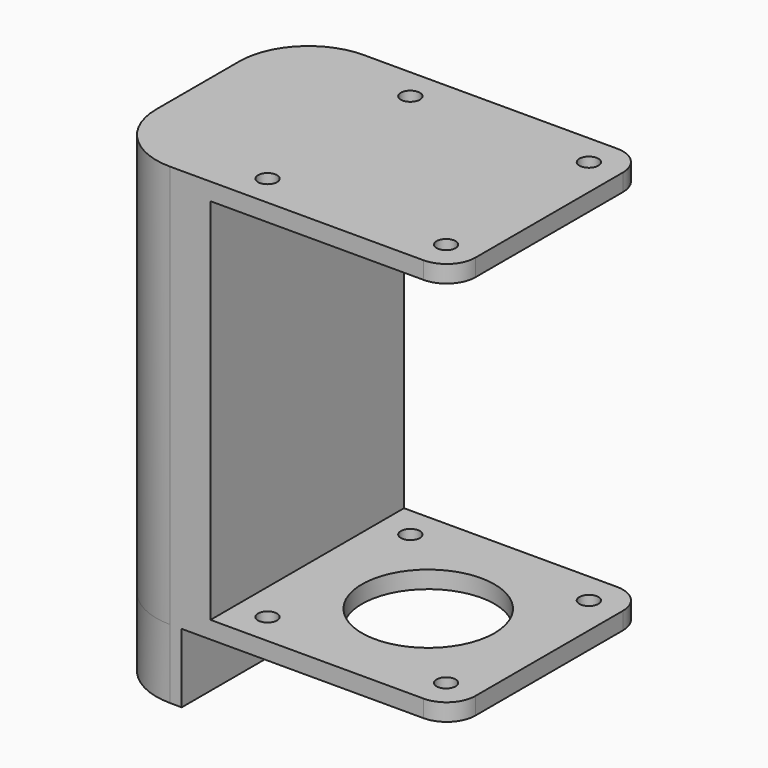
from build123d import *

# Parameters (mm, degrees)
F0_W      = 42
F0_H      = 42
F1_DEPTH  = 3
F2_R      = 11.5
F3_DEPTH  = 25
F4_W      = 42
F4_H      = 3
F4_H_2    = 67
F5_DEPTH  = 19
F6_W      = 42
F6_H      = 3
F7_DEPTH  = 42
F8_R      = 5
F9_D      = 3.3
F10_R     = 12
F12_DEPTH = 12
F14_DEPTH = 1


# Not quite as in the source:
# - a feature names something its author has since deleted; it is built from what else it names


with BuildPart() as f1:
    # F0 (on Top) → F1 (new body)
    with BuildSketch(Plane.XY):
        Rectangle(F0_W, F0_H)
    extrude(amount=F1_DEPTH)

    # F2 (on face) → F3 (cut)
    with BuildSketch(Plane(origin=(0, 0, 0), x_dir=(1, 0, 0), z_dir=(0, 0, -1))):
        Circle(F2_R)
    extrude(amount=-F3_DEPTH, mode=Mode.SUBTRACT)

    # F4 (on face) → F5 (join)
    with BuildSketch(Plane(origin=(-21, 0, 0), x_dir=(0, -1, 0), z_dir=(-1, 0, 0))):
        with Locations((0, 1.5)):
            Rectangle(F4_W, F4_H)
        with Locations((0, 36.5)):
            Rectangle(F4_W, F4_H_2)
    extrude(amount=F5_DEPTH)

    # F6 (on face) → F7 (join)
    with BuildSketch(Plane.YZ.offset(-21)):
        with Locations((0, 68.5)):
            Rectangle(F6_W, F6_H)
    extrude(amount=F7_DEPTH)

    # F8
    f8_edges = [f1.edges().sort_by_distance(p)[0] for p in [
        (21, 21, 1.5),
        (21, -21, 1.5),
        (21, -21, 68.5),
        (21, 21, 68.5),
    ]]
    fillet(f8_edges, radius=F8_R)

    # F9 (through all)
    with Locations(Plane(origin=(0, 0, 0), x_dir=(1, 0, 0), z_dir=(0, 0, -1))):
        with Locations((-15.5, -15.5), (15.5, -15.5), (15.5, 15.5), (-15.5, 15.5)):
            Hole(F9_D / 2)

    # F10
    f10_edges = [f1.edges().sort_by_distance(p)[0] for p in [
        (-40, -21, 35),
        (-40, 21, 35),
    ]]
    fillet(f10_edges, radius=F10_R)

    # F11 (on face) → F12 (join)
    with BuildSketch(Plane(origin=(0, 0, 0), x_dir=(1, 0, 0), z_dir=(0, 0, -1))):
        with BuildLine():
            Line((-26, -21), (-26, 21))
            Line((-26, 21), (-28, 21))
            ThreePointArc((-28, 21), (-36.4852813742, 17.4852813742), (-40, 9))
            Line((-40, 9), (-40, -9))
            ThreePointArc((-40, -9), (-36.4852813742, -17.4852813742), (-28, -21))
            Line((-28, -21), (-26, -21))
        make_face()
    extrude(amount=F12_DEPTH)

    # F13 (on face) → F14 (cut)
    with BuildSketch(Plane(origin=(0, 0, -12), x_dir=(1, 0, 0), z_dir=(0, 0, -1))):
        Polygon((-34.3291561734, 13.8271097128), (-34.3291561734, 13.8010392968), (-34.3163219754, 13.7125962563), (-34.2802923934, 13.6341532066), (-34.2247797128, 13.5694196654), (-34.1534948353, 13.5221079183), (-34.0701486625, 13.4959288669), (-33.9744900184, 13.4918830639), (-33.6002328215, 13.4918830639), (-32.9923355135, 13.4918830639), (-32.3260283508, 13.4918830639), (-31.7765408976, 13.4918830639), (-31.5191041022, 13.4918830639), (-31.7002456455, 13.3605228197), (-32.2358187745, 12.9783905954), (-32.9383236619, 12.477151783), (-33.6199622525, 11.9908008617), (-34.092935799, 11.6533336945), (-34.2138622028, 11.5664143172), (-34.2522084171, 11.5296983256), (-34.2834206772, 11.4874177114), (-34.3069654936, 11.4406069325), (-34.3223107603, 11.3902976792), (-34.3289257556, 11.3375257932), (-34.3291561734, 11.3008194889), (-34.3291561734, 11.2133846124), (-34.3291561734, 11.093462221), (-34.3291561734, 10.9735405215), (-34.3291561734, 10.8861056451), (-34.3284988255, 10.8410323404), (-34.3101892659, 10.7545011443), (-34.2695091207, 10.678789202), (-34.2101706756, 10.6176101828), (-34.1358848322, 10.5746756805), (-34.050363184, 10.5536972886), (-33.8706491234, 10.5522255213), (-33.2083116497, 10.5522255213), (-32.2537657549, 10.5522255213), (-31.2699997098, 10.5522255213), (-30.5199997098, 10.5522255213), (-30.2519789219, 10.5523908962), (-30.1644693154, 10.5679852632), (-30.0873617198, 10.6063619231), (-30.0243718803, 10.6638078983), (-29.9792148503, 10.7366102114), (-29.955606375, 10.8210579608), (-29.9530025855, 10.8704510788), (-29.9530025855, 10.9234865959), (-29.9530025855, 11.0043016334), (-29.9530025855, 11.0901678703), (-29.9530025855, 11.1583556015), (-29.9530025855, 11.1861365058), (-29.9658409352, 11.274569859), (-30.0018795125, 11.3530115248), (-30.0574025722, 11.4177478338), (-30.1286943692, 11.4650637326), (-30.21203985, 11.4912455518), (-30.3080562297, 11.4952927387), (-30.6852977859, 11.4952927387), (-31.2980428613, 11.4952927387), (-31.9696641626, 11.4952927387), (-32.5235330122, 11.4952927387), (-32.7830228088, 11.4952927387), (-32.6006191575, 11.6262302044), (-32.0613046814, 12.007134918), (-31.3538918273, 12.5067635742), (-30.6674912704, 12.9915513915), (-30.191212994, 13.3279349727), (-30.0694161233, 13.4145976383), (-30.0307197848, 13.4513419997), (-29.9992086043, 13.4937326331), (-29.9754278347, 13.5407212419), (-29.9599220367, 13.5912574532), (-29.953235771, 13.6442915864), (-29.9530025855, 13.6802755001), (-29.9530025855, 13.764942596), (-29.9530025855, 13.8810682846), (-29.9530025855, 13.9971946652), (-29.9530025855, 14.0818617612), (-29.9536599334, 14.1261538598), (-29.9719757205, 14.2126954351), (-30.012664861, 14.288412913), (-30.0720136852, 14.3495953918), (-30.1463050643, 14.39253197), (-30.2318239447, 14.4135103619), (-30.4115338536, 14.4149821292), (-31.0738713272, 14.4149821292), (-32.0284172221, 14.4149821292), (-33.0121839591, 14.4149821292), (-33.7621839591, 14.4149821292), (-34.0302054389, 14.4148167543), (-34.117720581, 14.3992216953), (-34.1948240249, 14.3608443435), (-34.2578048691, 14.3033956005), (-34.30295152, 14.2305877518), (-34.3265530758, 14.1461310072), (-34.3291561734, 14.0972921372), (-34.3291561734, 14.0475212172), (-34.3291561734, 13.971680573), (-34.3291561734, 13.8911001049), align=None)
        Polygon((-32.3764234053, 5.4123437425), (-32.1428005929, 5.4026316009), (-31.9076015295, 5.4119943102), (-31.6828113965, 5.440083822), (-31.4684281179, 5.4869022123), (-31.2644482342, 5.5524515567), (-31.0708689774, 5.6367332393), (-30.8876882718, 5.7397486438), (-30.7149026576, 5.8615012301), (-30.5525107509, 6.001992382), (-30.4038726373, 6.1579222132), (-30.2743619624, 6.3241717138), (-30.164045845, 6.5006813766), (-30.0729222092, 6.6874491257), (-30.0009869033, 6.8844721933), (-29.9482385434, 7.0917491955), (-29.9146736699, 7.3092780566), (-29.9002895149, 7.5370567006), (-29.9051123723, 7.7694139454), (-29.9292121286, 7.9925081209), (-29.9725950114, 8.2057102492), (-30.0352651722, 8.4090182542), (-30.1172260709, 8.6024293684), (-30.2184811671, 8.7859422076), (-30.3390339205, 8.9595546962), (-30.4788884829, 9.1232633744), (-30.6361772943, 9.2753113936), (-30.8040092734, 9.4089329143), (-30.9817422951, 9.5234602097), (-31.1693749756, 9.6188946636), (-31.3669059309, 9.6952383518), (-31.5743330853, 9.7524933502), (-31.7916543628, 9.7906617346), (-32.0188683795, 9.8097448889), (-32.254293709, 9.809718595), (-32.4828992274, 9.7904271652), (-32.701353911, 9.7518456896), (-32.9096591436, 9.693976244), (-33.1078135415, 9.6168202122), (-33.2958184885, 9.5203796701), (-33.4736732925, 9.4046566935), (-33.6413779538, 9.2696533584), (-33.7982751243, 9.1160110977), (-33.9376944531, 8.9503912671), (-34.0578950065, 8.7745610944), (-34.1588733246, 8.5885247313), (-34.2406259478, 8.3922884053), (-34.3031487243, 8.1858548842), (-34.3464381945, 7.9692303954), (-34.3704902066, 7.7424183987), (-34.3753040688, 7.5117128269), (-34.360955203, 7.3005567804), (-34.3274733628, 7.0966059583), (-34.2748557806, 6.8998672801), (-34.2031017643, 6.7103469734), (-34.1122078543, 6.5280519575), (-34.0021733585, 6.35298846), (-33.8729962012, 6.1851634003), (-33.7247441929, 6.0246605039), (-33.5628484109, 5.8788213082), (-33.3907208365, 5.7524472205), (-33.2083545503, 5.6455327053), (-33.0157467845, 5.5580715349), (-32.8128920035, 5.490057482), (-32.5997860556, 5.4414829351), align=None)
        Polygon((-33.4991237257, 7.4768816938), (-33.5027460584, 7.6090044615), (-33.4947935332, 7.7410372763), (-33.4759456403, 7.8664730864), (-33.4461996118, 7.9853056643), (-33.4055540639, 8.0975322421), (-33.3540062288, 8.2031472845), (-33.2915547227, 8.3021466396), (-33.2181967776, 8.3945254639), (-33.1339296259, 8.4802796056), (-33.0401980489, 8.5581379617), (-32.939166451, 8.6259651894), (-32.8308555906, 8.6837329191), (-32.7152661594, 8.7314439186), (-32.5923967737, 8.7691030314), (-32.4622488174, 8.7967137172), (-32.3248209066, 8.8142815117), (-32.1801144251, 8.8218084906), (-32.0304051804, 8.8192406823), (-31.8869573471, 8.8064334702), (-31.7508358286, 8.7833813188), (-31.6220371653, 8.750083536), (-31.5005599731, 8.706540814), (-31.3864007926, 8.6527517687), (-31.2795582396, 8.588717784), (-31.1800288545, 8.5144381681), (-31.0886222131, 8.4306173209), (-31.0083870256, 8.3401046727), (-30.9396146008, 8.2431963757), (-30.8823049388, 8.1398868945), (-30.8364573475, 8.0301686176), (-30.802072519, 7.9140367015), (-30.7791497613, 7.7914835347), (-30.7676883825, 7.6625042737), (-30.767706373, 7.5319017095), (-30.7793151362, 7.4085728722), (-30.8025354303, 7.2906799558), (-30.8373679473, 7.1782278038), (-30.8838161469, 7.0712205679), (-30.941882105, 6.9696630917), (-31.0115672054, 6.8735602189), (-31.0928749078, 6.782916101), (-31.1853893533, 6.6980829382), (-31.2850190704, 6.6226913665), (-31.3907226817, 6.5577052653), (-31.5024974195, 6.5031211751), (-31.6203391319, 6.4589384038), (-31.7442436675, 6.4251548756), (-31.8742082584, 6.4017678227), (-32.0102294448, 6.3887765532), (-32.1539388334, 6.3861720718), (-32.3005384767, 6.3938201411), (-32.4402781762, 6.4116647137), (-32.5731572399, 6.4397057894), (-32.699172208, 6.4779433683), (-32.8183230807, 6.5263774503), (-32.9306077819, 6.5850080356), (-33.036024928, 6.6538351241), (-33.1345364618, 6.7328310379), (-33.2229760425, 6.8197386521), (-33.2992948207, 6.9131111096), (-33.3634941802, 7.0129463344), (-33.415575505, 7.1192436346), (-33.455539487, 7.2319995505), (-33.4833888939, 7.3512126982), align=None, mode=Mode.SUBTRACT)
        Polygon((-34.1037571286, 1.8411790328), (-34.0199999404, 1.8296982794), (-33.731121851, 1.8296982794), (-33.0121839591, 1.8296982794), (-32.0847318671, 1.8296982794), (-31.1703118693, 1.8296982794), (-30.4904702602, 1.8296982794), (-30.2519789219, 1.8298636543), (-30.1690928927, 1.843962728), (-30.0953004061, 1.8785696708), (-30.0337325138, 1.9305561991), (-29.9875181917, 1.9967954129), (-29.9597884912, 2.0741583362), (-29.9530025855, 2.140396858), (-29.9530025855, 2.1758507417), (-29.9530025855, 2.2439858851), (-29.9530025855, 2.3256437117), (-29.9530025855, 2.4016670294), (-29.9530025855, 2.4528979536), (-29.9544750447, 2.4941870104), (-29.9736834411, 2.5752096315), (-30.012664861, 2.6463962528), (-30.0682896366, 2.7046213582), (-30.1374281004, 2.746755972), (-30.2169485086, 2.769674578), (-30.2873387011, 2.7729606254), (-30.4784317991, 2.7729606254), (-30.789516483, 2.7729606254), (-31.1389985852, 2.7729606254), (-31.4452839378, 2.7729606254), (-31.6267776812, 2.7729606254), (-31.6461729027, 2.7920949836), (-31.6461729027, 2.8167524477), (-31.6461729027, 2.8436303637), (-31.6461729027, 2.8788842752), (-31.5843365358, 2.921018889), (-31.3295208284, 3.0914601931), (-30.9613942652, 3.3376916294), (-30.57168455, 3.5983605004), (-30.2521200787, 3.8121106492), (-30.0944271713, 3.9175879945), (-30.0563369768, 3.9466496892), (-30.0209149225, 3.9839988106), (-29.9923638833, 4.0263797568), (-29.9711931306, 4.0728424873), (-29.9579084764, 4.1224376532), (-29.9530178083, 4.1742152141), (-29.9530025855, 4.2005554887), (-29.9530025855, 4.2636539636), (-29.9530025855, 4.3467282019), (-29.9530025855, 4.4298024403), (-29.9530025855, 4.4929009151), (-29.953084927, 4.5235388608), (-29.9778150453, 4.6389117131), (-30.0395939809, 4.7311417692), (-30.1281996284, 4.7947792693), (-30.2334098829, 4.8243779135), (-30.345002639, 4.8144893259), (-30.4380242803, 4.7704608583), (-30.574143723, 4.6790985014), (-30.8499883342, 4.4939512878), (-31.1863816026, 4.2681647538), (-31.5041449408, 4.0548830519), (-31.7240997614, 3.9072496425), (-31.7985212261, 3.9177519855), (-31.8759228984, 4.0642374578), (-31.9623641416, 4.1936664832), (-32.0578511833, 4.3060259145), (-32.162390251, 4.4013039888), (-32.2759868802, 4.479488943), (-32.3977415423, 4.5411689304), (-32.5197812858, 4.5915155487), (-32.6402828353, 4.6317230954), (-32.7592489586, 4.6617964139), (-32.8766858832, 4.6817417318), (-32.9925963768, 4.6915625087), (-33.1507944042, 4.6895876974), (-33.3368169283, 4.6668524568), (-33.5087735923, 4.622033096), (-33.6666685476, 4.5551309989), (-33.8105080219, 4.4661468573), (-33.9402961668, 4.3550834392), (-34.0547826374, 4.2232125395), (-34.1496040279, 4.0750491002), (-34.2243915316, 3.9109868381), (-34.2791506839, 3.7310195256), (-34.3138856367, 3.5351409352), (-34.3286026173, 3.3233469153), (-34.3291561734, 3.2187656389), (-34.3291561734, 3.0266180166), (-34.3291561734, 2.7559318561), (-34.3291561734, 2.4734660221), (-34.3291561734, 2.2459759192), (-34.3291561734, 2.1402197201), (-34.320171958, 2.0645811239), (-34.2901131703, 1.9883647536), (-34.2419406435, 1.9236402077), (-34.1787798936, 1.8735357701), align=None)
        Polygon((-33.5022104929, 2.7795756206), (-33.5492966659, 2.7795756206), (-33.5492966659, 2.8123122359), (-33.5492966659, 2.846046636), (-33.5492966659, 2.8849713164), (-33.5492966659, 2.9242952491), (-33.5492966659, 2.9592274062), (-33.5492966659, 2.9967543574), (-33.5477868417, 3.0650894729), (-33.5419890335, 3.1426841979), (-33.5318430424, 3.2158207205), (-33.5173474842, 3.2844976569), (-33.498503051, 3.348714315), (-33.4753097427, 3.4084679272), (-33.4477661756, 3.4637584934), (-33.4158730414, 3.5145839378), (-33.3799223411, 3.5606647146), (-33.3408648073, 3.6010466314), (-33.2987696344, 3.6356549581), (-33.2536312869, 3.6644903868), (-33.205446305, 3.6875543014), (-33.1542091533, 3.7048501614), (-33.099914988, 3.7163786589), (-33.0425603496, 3.7221418698), (-32.9411170443, 3.7200916364), (-32.8114569093, 3.6979265586), (-32.6998932148, 3.653595711), (-32.6064259609, 3.5870984018), (-32.5310516878, 3.4984318631), (-32.4737703955, 3.3875967868), (-32.4345793162, 3.2545917891), (-32.4134777581, 3.0994147941), (-32.4094582489, 2.9691028468), (-32.4094582489, 2.9431888104), (-32.4094582489, 2.9094059742), (-32.4094582489, 2.8722519813), (-32.4094582489, 2.8362217073), (-32.4094582489, 2.8058107196), (-32.4108628975, 2.7795756206), (-32.4725982405, 2.7795756206), (-32.6075780495, 2.7795756206), (-32.7906895606, 2.7795756206), (-32.9968213937, 2.7795756206), (-33.2008607848, 2.7795756206), (-33.3776942778, 2.7795756206), align=None, mode=Mode.SUBTRACT)
        Polygon((-34.3291561734, -1.2968889273), (-34.3291561734, -1.4208239085), (-34.3213088238, -1.4903464018), (-34.2989313189, -1.5543188033), (-34.263769436, -1.6109946436), (-34.2175703366, -1.6586288371), (-34.1620784144, -1.6954742225), (-34.0990415227, -1.7197850221), (-34.0302054389, -1.7298154584), (-34.0076168907, -1.7299801414), (-33.9677656958, -1.7299801414), (-33.91032664, -1.7299801414), (-33.8455591936, -1.7299801414), (-33.7837235185, -1.7299801414), (-33.7350777012, -1.7299801414), (-33.7098825958, -1.7299801414), (-33.6582849406, -1.7259343383), (-33.5925563824, -1.7075299822), (-33.5336220332, -1.6758423557), (-33.4832297465, -1.6326186203), (-33.4431252997, -1.5796038616), (-33.4150551623, -1.518544549), (-33.4007671876, -1.451187152), (-33.3992954204, -1.4083294556), (-33.3992954204, -1.3356503087), (-33.3992954204, -1.2177006527), (-33.3992954204, -1.0771153963), (-33.3992954204, -0.9365301399), (-33.3992954204, -0.8185797921), (-33.3992954204, -0.7459006452), (-33.3667698484, -0.7334061923), (-33.0730356882, -0.7334061923), (-32.5579469024, -0.7334061923), (-31.9248025931, -0.7334061923), (-31.2769011704, -0.7334061923), (-30.7175410443, -0.7334061923), (-30.3500220089, -0.7334061923), (-30.2418578408, -0.7327488444), (-30.1737469155, -0.7205713024), (-30.1116794389, -0.6943624973), (-30.0574025722, -0.6558668229), (-30.012664861, -0.6068307486), (-29.9792148503, -0.5490000519), (-29.9588003936, -0.4841205103), (-29.9530025855, -0.4238375601), (-29.9530025855, -0.4019298859), (-29.9530025855, -0.3540389807), (-29.9530025855, -0.2908636999), (-29.9530025855, -0.2231028989), (-29.9530025855, -0.1614561249), (-29.9530025855, -0.0993000793), (-29.9608520109, -0.029776894), (-29.9832357434, 0.0341989672), (-30.0184059296, 0.0908796512), (-30.0646133323, 0.1385186883), (-30.1201100981, 0.1753689173), (-30.1831483737, 0.1996838685), (-30.2519789219, 0.2097149968), (-30.3868646264, 0.2098803717), (-30.7881139103, 0.2098803717), (-31.3664464794, 0.2098803717), (-32.0185646156, 0.2098803717), (-32.641168525, 0.2098803717), (-33.1309591055, 0.2098803717), (-33.384638639, 0.2098803717), (-33.3992954204, 0.2293129583), (-33.3992954204, 0.310617201), (-33.3992954204, 0.4343618973), (-33.3992954204, 0.5776941758), (-33.3992954204, 0.7177618572), (-33.3992954204, 0.8317127623), (-33.3992954204, 0.8966940198), (-33.4018985179, 0.944194668), (-33.4182623279, 1.0107618637), (-33.4481578165, 1.0707825667), (-33.4898392062, 1.1225109994), (-33.5415586437, 1.1641986167), (-33.6015710433, 1.1940996408), (-33.6681278599, 1.2104662186), (-33.711657435, 1.213070008), (-33.7408305329, 1.213070008), (-33.7919888029, 1.213070008), (-33.8548713909, 1.213070008), (-33.9192202106, 1.213070008), (-33.9747744079, 1.213070008), (-34.0112758965, 1.213070008), (-34.040327904, 1.2124126602), (-34.1084429809, 1.2002337343), (-34.1705083817, 1.1740214695), (-34.2247797128, 1.1355230273), (-34.2695091207, 1.0864848771), (-34.30295152, 1.0286548723), (-34.3233604411, 0.9637794824), (-34.3291561734, 0.9011369994), (-34.3291561734, 0.7443955166), (-34.3291561734, 0.401751216), (-34.3291561734, -0.0502473982), (-34.3291561734, -0.5350525142), (-34.3291561734, -0.9761156279), align=None)
        Polygon((-34.3291561734, -5.4243000101), (-34.3291561734, -5.4537692605), (-34.3148944926, -5.5468573285), (-34.2750183877, -5.6285822738), (-34.2138940323, -5.694576539), (-34.1358848322, -5.7404718745), (-34.0453569611, -5.7619007227), (-33.8829678222, -5.7629254934), (-33.3650005447, -5.7629254934), (-32.6577406105, -5.7629254934), (-31.9727502378, -5.7629254934), (-31.5215923368, -5.7629254934), (-31.3504376373, -5.7595529529), (-31.1437889212, -5.7302781391), (-30.9408718651, -5.6709230873), (-30.7417037676, -5.5814725747), (-30.5463005435, -5.4619113786), (-30.3553707446, -5.3121426267), (-30.1904656933, -5.1290497981), (-30.0618019593, -4.9110642533), (-29.9693691633, -4.6581873762), (-29.9131555423, -4.3704219345), (-29.8931493332, -4.0477679283), (-29.8999995899, -3.8541097897), (-29.9222656917, -3.6753063289), (-29.9599365675, -3.5033579683), (-30.0130308999, -3.3382723193), (-30.0815673714, -3.1800563015), (-30.1650560849, -3.0306155315), (-30.2621982593, -2.8957997134), (-30.3729364632, -2.776028166), (-30.4972727726, -2.6713071168), (-30.6352127228, -2.5816434852), (-30.7853717318, -2.5069424746), (-30.9361036713, -2.4463516089), (-31.0847853775, -2.399692366), (-31.2314189261, -2.3669772011), (-31.3760036253, -2.3482213368), (-31.5028496195, -2.343264242), (-31.808884488, -2.343264242), (-32.4210490215, -2.343264242), (-33.1316123017, -2.343264242), (-33.7328441024, -2.343264242), (-34.0170121215, -2.343264242), (-34.1037571286, -2.3547429195), (-34.1868867225, -2.392128022), (-34.2547395523, -2.4512222105), (-34.30295152, -2.5276593113), (-34.3271585278, -2.6170752266), (-34.3291561734, -2.6646755148), (-34.3291561734, -2.7229462886), (-34.3291561734, -2.8065962253), (-34.3291561734, -2.890246162), (-34.3291561734, -2.9485162438), (-34.3271585278, -2.996117224), (-34.30295152, -3.0855331393), (-34.2547395523, -3.1619702401), (-34.1868867225, -3.2210637366), (-34.1037571286, -3.2584488392), (-34.0172529184, -3.2699275166), (-33.7559792873, -3.2699275166), (-33.2031871042, -3.2699275166), (-32.5498719029, -3.2699275166), (-31.9870278332, -3.2699275166), (-31.7056497369, -3.2699275166), (-31.5710062132, -3.2753800441), (-31.4309150056, -3.2960242266), (-31.3044149839, -3.3320600361), (-31.1915192951, -3.38349716), (-31.0922410861, -3.4503439015), (-31.007058491, -3.5321657192), (-30.938087478, -3.6267705309), (-30.8855909861, -3.7338670277), (-30.849574551, -3.8534628211), (-30.8300437083, -3.9855634465), (-30.8269991498, -4.1230806183), (-30.840359918, -4.2433302997), (-30.8700921075, -4.354190286), (-30.9161901829, -4.4556591932), (-30.9786486085, -4.5477384053), (-31.0574521616, -4.6304258463), (-31.1494178947, -4.7007606831), (-31.2519724638, -4.7561474297), (-31.365115177, -4.7965957732), (-31.4888453424, -4.8221133251), (-31.623162268, -4.8327097726), (-31.7965962348, -4.8330405223), (-32.2876558426, -4.8330405223), (-32.9427908595, -4.8330405223), (-33.5671619968, -4.8330405223), (-33.9659285815, -4.8330405223), (-34.0701486625, -4.8370863254), (-34.1578056533, -4.8653737336), (-34.2317946523, -4.9169769243), (-34.2877508697, -4.9875324916), (-34.3213088238, -5.072674262), (-34.3291561734, -5.1444552641), (-34.3291561734, -5.1874222878), (-34.3291561734, -5.265481308), (-34.3291561734, -5.3529895306), align=None)
        Polygon((-34.3291561734, -8.5249925549), (-34.3291561734, -8.7168633992), (-34.3133964315, -8.8145736605), (-34.2695091207, -8.8994393447), (-34.2025869572, -8.96636566), (-34.117720581, -9.0102571224), (-34.0199999404, -9.0260196321), (-33.6291872648, -9.0260196321), (-32.6972486006, -9.0260196321), (-31.5849343763, -9.0260196321), (-30.6529957122, -9.0260196321), (-30.2621830365, -9.0260196321), (-30.1644693154, -9.0102571224), (-30.0795980956, -8.96636566), (-30.012664861, -8.8994393447), (-29.968767171, -8.8145736605), (-29.9530025855, -8.7168633992), (-29.9530025855, -8.5249925549), (-29.9530025855, -8.0674556119), (-29.9530025855, -7.5213628414), (-29.9530025855, -7.0638252066), (-29.9530025855, -6.8719550542), (-29.968767171, -6.7742337217), (-30.012664861, -6.68936181), (-30.0795980956, -6.622432727), (-30.1644693154, -6.5785405726), (-30.2621830365, -6.562777371), (-30.2880015845, -6.562777371), (-30.3495680929, -6.562777371), (-30.4230505881, -6.562777371), (-30.4846170964, -6.562777371), (-30.5104356444, -6.562777371), (-30.60814383, -6.5785405726), (-30.6930032867, -6.622432727), (-30.7599219905, -6.68936181), (-30.8038072254, -6.7742337217), (-30.8195676593, -6.8719550542), (-30.8195676593, -6.9978759178), (-30.8195676593, -7.2981489594), (-30.8195676593, -7.6565391629), (-30.8195676593, -7.9568122044), (-30.8195676593, -8.0827330681), (-30.9138458729, -8.0827330681), (-31.1386643757, -8.0827330681), (-31.4069958469, -8.0827330681), (-31.6318136578, -8.0827330681), (-31.7260925633, -8.0827330681), (-31.7260925633, -7.9568122044), (-31.7260925633, -7.6565391629), (-31.7260925633, -7.2981489594), (-31.7260925633, -6.9978759178), (-31.7260925633, -6.8719550542), (-31.741855073, -6.7742337217), (-31.7857465354, -6.68936181), (-31.8526721587, -6.622432727), (-31.9375378429, -6.5785405726), (-32.0352487962, -6.562777371), (-32.0596931412, -6.562777371), (-32.1179846734, -6.562777371), (-32.1875590625, -6.562777371), (-32.2458505947, -6.562777371), (-32.2702949397, -6.562777371), (-32.3680176561, -6.5785405726), (-32.4528909517, -6.622432727), (-32.5198200347, -6.68936181), (-32.563712881, -6.7742337217), (-32.5794760826, -6.8719550542), (-32.5794760826, -6.9978759178), (-32.5794760826, -7.2981489594), (-32.5794760826, -7.6565391629), (-32.5794760826, -7.9568122044), (-32.5794760826, -8.0827330681), (-32.6713221092, -8.0827330681), (-32.89034142, -8.0827330681), (-33.1517506723, -8.0827330681), (-33.3707692912, -8.0827330681), (-33.4626153177, -8.0827330681), (-33.4626153177, -7.9568122044), (-33.4626153177, -7.6565391629), (-33.4626153177, -7.2981489594), (-33.4626153177, -6.9978759178), (-33.4626153177, -6.8719550542), (-33.4783757515, -6.7742337217), (-33.5222609864, -6.68936181), (-33.5891796903, -6.622432727), (-33.674039147, -6.5785405726), (-33.7717473325, -6.562777371), (-33.7975658805, -6.562777371), (-33.8591323889, -6.562777371), (-33.9326148841, -6.562777371), (-33.9941820844, -6.562777371), (-34.0199999404, -6.562777371), (-34.117720581, -6.5785405726), (-34.2025869572, -6.622432727), (-34.2695091207, -6.68936181), (-34.3133964315, -6.7742337217), (-34.3291561734, -6.8719550542), (-34.3291561734, -7.0638252066), (-34.3291561734, -7.5213628414), (-34.3291561734, -8.0674556119), align=None)
        Polygon((-34.3291561734, -10.5007463368), (-34.3291561734, -10.5268859473), (-34.3163378901, -10.6152044377), (-34.2803546684, -10.6935416198), (-34.2249139501, -10.7581893597), (-34.1537238691, -10.8054402157), (-34.0704925592, -10.8315860537), (-33.9748975741, -10.8356270132), (-33.6005781021, -10.8356270132), (-32.9925804621, -10.8356270132), (-32.3261625881, -10.8356270132), (-31.7765837982, -10.8356270132), (-31.5191047941, -10.8356270132), (-31.7002574086, -10.9669955607), (-32.2358644428, -11.349152003), (-32.9384143067, -11.8504233368), (-33.6200957979, -12.3368047038), (-34.09309979, -12.6742940132), (-34.2140116629, -12.7612085469), (-34.2523039055, -12.7978864815), (-34.2834746489, -12.8401172757), (-34.3069904036, -12.8868692392), (-34.3223183717, -12.937109298), (-34.3289257556, -12.9898064539), (-34.3291561734, -13.0265259052), (-34.3291561734, -13.1140714929), (-34.3291561734, -13.2341454203), (-34.3291561734, -13.3542186558), (-34.3291561734, -13.4417642434), (-34.3284995174, -13.4868451595), (-34.310212792, -13.5732760236), (-34.2695852347, -13.648898013), (-34.2103242874, -13.710003686), (-34.1361380841, -13.7528862924), (-34.0507347585, -13.7738390824), (-33.8710324609, -13.7753087738), (-33.2085524466, -13.7753087738), (-32.2538024279, -13.7753087738), (-31.2698253396, -13.7753087738), (-30.5196641164, -13.7753087738), (-30.2516004279, -13.7751440908), (-30.1641946132, -13.7595684063), (-30.087183198, -13.7212387988), (-30.024275008, -13.663862018), (-29.9791788692, -13.5911455061), (-29.9556029153, -13.5067960129), (-29.9530025855, -13.4574284969), (-29.9530025855, -13.4042691216), (-29.9530025855, -13.3232644911), (-29.9530025855, -13.2371975902), (-29.9530025855, -13.1688500197), (-29.9530025855, -13.1410047645), (-29.9658229446, -13.0526745111), (-30.0018130857, -12.974324874), (-30.0572627993, -12.9096660629), (-30.1284639515, -12.8624069036), (-30.2117077163, -12.8362562219), (-30.3076728921, -12.8322145705), (-30.6849725717, -12.8322145705), (-31.2978124436, -12.8322145705), (-31.9695375366, -12.8322145705), (-32.5234928794, -12.8322145705), (-32.7830228088, -12.8322145705), (-32.6006094703, -12.7012701854), (-32.0612652405, -12.3203460973), (-31.3538143294, -11.8206932231), (-30.6673764075, -11.3358811877), (-30.1910725292, -10.9994809998), (-30.0692867296, -10.9128245617), (-30.0306353675, -10.8761237929), (-29.9991594762, -10.8337898989), (-29.9754043086, -10.786866333), (-29.9599144253, -10.7363965484), (-29.9532350791, -10.6834226144), (-29.9530025855, -10.6474186344), (-29.9530025855, -10.5626366755), (-29.9530025855, -10.4463532234), (-29.9530025855, -10.3300697713), (-29.9530025855, -10.2452871205), (-29.9536592414, -10.2009887944), (-29.9719494266, -10.114562082), (-30.0125839034, -10.038947012), (-30.0718545379, -9.9778475665), (-30.1460525043, -9.9349711876), (-30.2314682849, -9.9140218574), (-30.411175426, -9.9125521659), (-31.0736547484, -9.9125521659), (-32.028405459, -9.9125521659), (-33.0123825473, -9.9125521659), (-33.7625437706, -9.9125521659), (-34.0306060751, -9.9127168489), (-34.1179987429, -9.9282904575), (-34.1949977032, -9.9666145296), (-34.2578955139, -10.0239843908), (-34.3029847333, -10.0966939833), (-34.3265565356, -10.1810386329), (-34.3291561734, -10.2298470573), (-34.3291561734, -10.2797494469), (-34.3291561734, -10.355791447), (-34.3291561734, -10.4365857262), align=None)
    extrude(amount=-F14_DEPTH, mode=Mode.SUBTRACT)


solid = f1.part
